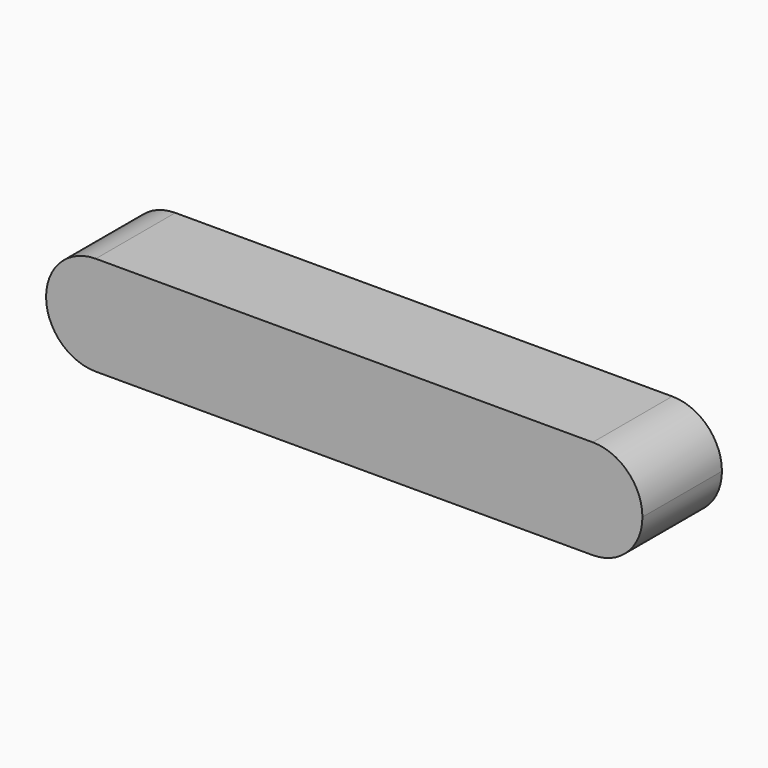
from build123d import *

# Parameters (mm, degrees)
F0_W     = 30
F0_H     = 5
F1_DEPTH = 5
F2_R     = 2.49999


# Not quite as in the source:
# - a fillet or chamfer is up to 0.001 mm smaller than in the source, because OpenCascade refuses the exact size


with BuildPart() as f1:
    # F0 (on Top) → F1 (new body)
    with BuildSketch(Plane.XY):
        Rectangle(F0_W, F0_H)
    extrude(amount=F1_DEPTH)

    # F2 (radius 2.5 in the source; OpenCascade refuses exactly that, so slightly less here)
    f2_edges = [f1.edges().sort_by_distance(p)[0] for p in [
        (-15, 0, 5),
        (-15, 0, 0),
        (15, 0, 5),
        (15, 0, 0),
    ]]
    fillet(f2_edges, radius=F2_R)


solid = f1.part
